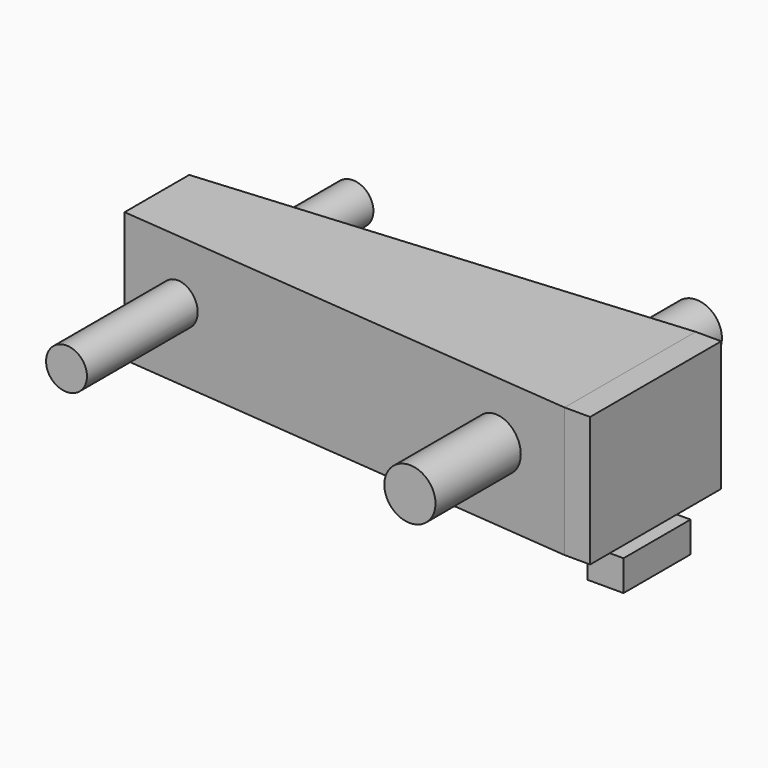
from build123d import *

# Parameters (mm, degrees)
F0_W           = 92.7798543125
F0_H           = 32.0377349854
F1_DEPTH       = 25.4
F3_DEPTH       = 25
F4_DEPTH       = 25
F6_E4_LEFT_W   = 16.385298688
F6_E4_LEFT_H   = 6
F7_DEPTH       = 7
F8_DEPTH       = 5
F9_R           = 5
F9_R_2         = 4
F10_DEPTH      = 50
F10_DEPTH_BACK = 20


with BuildPart() as f1:
    # F0 (on Top) → F1 (new body)
    with BuildSketch(Plane.XY):
        with Locations((26.091161184, 16.0188674927)):
            Rectangle(F0_W, F0_H)
    extrude(amount=F1_DEPTH)

    # F2 (on face) → F3 (cut)
    with BuildSketch(Plane.XY.offset(25.4)):
        Polygon((-20.2987659723, 24.2482833564), (72.4810883403, 32.0377349854), (-20.2987659723, 32.0377349854), align=None)
        Polygon((-20.2987659723, 0), (72.4810883403, 0), (-20.2987659723, 8.4725329652), align=None)
    extrude(amount=-F3_DEPTH, mode=Mode.SUBTRACT)

    # F4 (cut): faces of the model
    f4_faces = [f1.faces().sort_by_distance(p)[0] for p in [
        (10.6278521319, 29.441251109, 0.4),
        (10.6278521319, 2.8241776551, 0.4),
    ]]
    extrude(f4_faces, amount=-F4_DEPTH, mode=Mode.SUBTRACT)


with BuildPart() as f7:
    # F6_E4_left (on explicit) → F7 (new body)
    with BuildSketch(Plane(origin=(73.1688588858, 4.8025916331, 0), x_dir=(0, 1, 0), z_dir=(-1, 0, 0))):
        with Locations((8.192649344, 3)):
            Rectangle(F6_E4_LEFT_W, F6_E4_LEFT_H)
    extrude(amount=-F7_DEPTH)


with BuildPart() as f8:
    # F8 (new): a face of the model
    f8_faces = [f1.part.faces().sort_by_distance(p)[0] for p in [
        (72.4810883403, 16.0188674927, 12.7),
    ]]
    extrude(f8_faces, amount=F8_DEPTH)


with BuildPart() as f1_1:
    add(f1.part)

    # F9 (on Front) → F10 (join, two sides)
    with BuildSketch(Plane.XZ) as f10_sk:
        with Locations((58.2476481795, 14)):
            Circle(F9_R)
        with Locations((-8.8881440461, 13.738758862)):
            Circle(F9_R_2)
    extrude(amount=-F10_DEPTH)
    extrude(f10_sk.sketch, amount=F10_DEPTH_BACK)


solid = Compound([f7.part, f8.part, f1_1.part])
